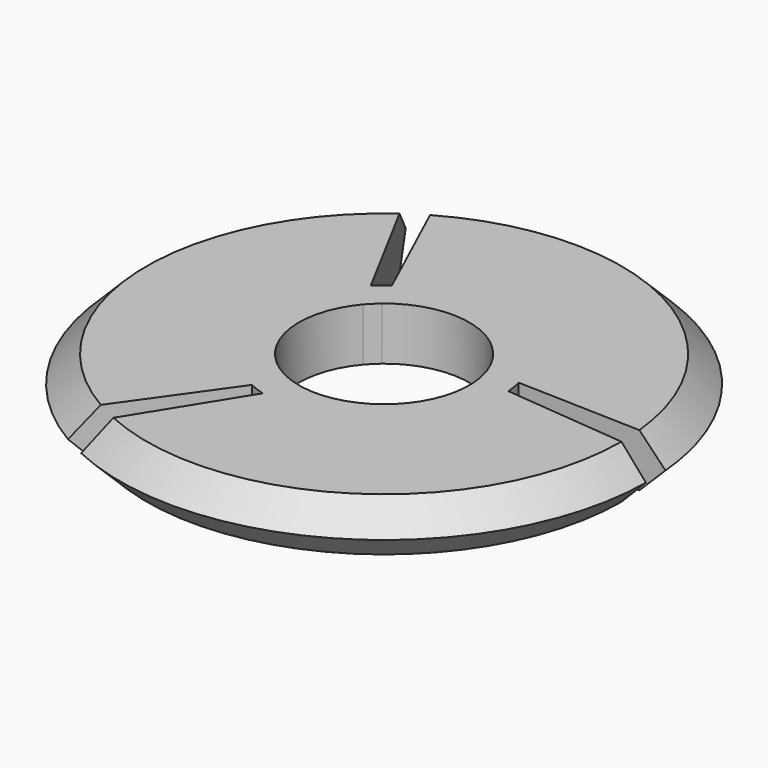
from build123d import *

# Parameters (mm, degrees)
F1_DEPTH     = 7
F2_T2_ANGLE  = 147.8228871573
F2_T4_ANGLE  = 147.8228871573
F2_T6_ANGLE  = 147.8228871573
F2_T8_ANGLE  = 147.8228871573
F2_T10_ANGLE = 147.8228871573
F2_T12_ANGLE = 147.8228871573


# Not quite as in the source:
# - a fillet or chamfer that OpenCascade refuses, or shapes differently, is made with other operations: its cross-section is extruded or revolved along the edge and cut away or added


with BuildPart() as f1:
    # F0 (on Top) → F1 (new body)
    with BuildSketch(Plane.XY):
        with BuildLine():
            Line((-28.4060324401, -36.6326823344), (-16.7057452382, -20.1458706432))
            ThreePointArc((-16.7057452382, -20.1458706432), (-25.4681782111, -8.7912963767), (-20.97968548, 4.8307453711))
            Line((-20.97968548, 4.8307453711), (-30.6144689612, 22.7902857677))
            ThreePointArc((-30.6144689612, 22.7902857677), (-45.7201890255, -7.5236357069), (-28.4060324401, -36.6326823344))
        make_face()
        with BuildLine():
            ThreePointArc((-19.29435824, 6.2304415143), (-5.0797919896, 8.1416439346), (4.4729958499, -2.5565256692))
            Line((4.4729958499, -2.5565256692), (24.8438058142, -3.1923286128))
            ThreePointArc((24.8438058142, -3.1923286128), (6.144039761, 25.0465694426), (-27.722212391, 24.6065933083))
            Line((-27.722212391, 24.6065933083), (-19.29435824, 6.2304415143))
        make_face()
        with BuildLine():
            ThreePointArc((4.9156669829, -6.2104463577), (-1.1968722093, -18.4456132191), (-14.6509092006, -20.9055587751))
            Line((-14.6509092006, -20.9055587751), (-25.3869356838, -38.229296228))
            ThreePointArc((-25.3869356838, -38.229296228), (8.4185504337, -36.154272809), (24.9706460004, -6.6052500471))
            Line((24.9706460004, -6.6052500471), (4.8425046474, -4.7159099443))
            ThreePointArc((4.8425046474, -4.7159099443), (4.8973654542, -5.4622833042), (4.9156669829, -6.2104463577))
        make_face()
        with BuildLine():
            Line((-16.7057452382, -20.1458706432), (-14.3009175091, -16.7572408399))
            ThreePointArc((-14.3009175091, -16.7572408399), (-21.2699622014, -9.0563128177), (-18.9622633915, 1.0702069463))
            Line((-18.9622633915, 1.0702069463), (-20.97968548, 4.8307453711))
            ThreePointArc((-20.97968548, 4.8307453711), (-25.4681782111, -8.7912963767), (-16.7057452382, -20.1458706432))
        make_face()
        with BuildLine():
            ThreePointArc((-17.5621326109, 2.4534847075), (-7.4084109648, 4.63839044), (0.2075629978, -2.4233952356))
            Line((0.2075629978, -2.4233952356), (4.4729958499, -2.5565256692))
            ThreePointArc((4.4729958499, -2.5565256692), (-5.0797919896, 8.1416439346), (-19.29435824, 6.2304415143))
            Line((-19.29435824, 6.2304415143), (-17.5621326109, 2.4534847075))
        make_face()
        with BuildLine():
            ThreePointArc((0.7054512892, -4.3275829408), (-2.4792256646, -14.2134166955), (-12.4028984371, -17.2781507839))
            Line((-12.4028984371, -17.2781507839), (-14.6509092006, -20.9055587751))
            ThreePointArc((-14.6509092006, -20.9055587751), (-1.1968722093, -18.4456132191), (4.9156669829, -6.2104463577))
            ThreePointArc((4.9156669829, -6.2104463577), (4.8973654542, -5.4622833042), (4.8425046474, -4.7159099443))
            Line((4.8425046474, -4.7159099443), (0.7054512892, -4.3275829408))
        make_face()
        with BuildLine():
            Line((-20.97968548, 4.8307453711), (-18.9622633915, 1.0702069463))
            ThreePointArc((-18.9622633915, 1.0702069463), (-18.2773306397, 1.7771628324), (-17.5621326109, 2.4534847075))
            Line((-17.5621326109, 2.4534847075), (-19.29435824, 6.2304415143))
            ThreePointArc((-19.29435824, 6.2304415143), (-20.1621039238, 5.5607939156), (-20.97968548, 4.8307453711))
        make_face()
        with BuildLine():
            ThreePointArc((0.2075629978, -2.4233952356), (0.4773383786, -3.3700423415), (0.7054512892, -4.3275829408))
            Line((0.7054512892, -4.3275829408), (4.8425046474, -4.7159099443))
            ThreePointArc((4.8425046474, -4.7159099443), (4.6964456573, -3.6295963387), (4.4729958499, -2.5565256692))
            Line((4.4729958499, -2.5565256692), (0.2075629978, -2.4233952356))
        make_face()
        with BuildLine():
            Line((-14.6509092006, -20.9055587751), (-12.4028984371, -17.2781507839))
            Line((-12.4028984371, -17.2781507839), (-14.3009175091, -16.7572408399))
            Line((-14.3009175091, -16.7572408399), (-16.7057452382, -20.1458706432))
            ThreePointArc((-16.7057452382, -20.1458706432), (-15.6919405642, -20.56253665), (-14.6509092006, -20.9055587751))
        make_face()
    extrude(amount=F1_DEPTH)

    # F2: chamfer of 4 on 6 edges, made by hand

    # F2_s1 → F2_t2 (revolve, cut)
    with BuildSketch(Plane(origin=(-11.2150452206, -3.6909975733, 0), x_dir=(0, 0, 1), z_dir=(0.9498795724, 0.3126160553, 0))):
        Polygon((3, -32.7063288851), (7, -28.7063288851), (7, -32.7063288851), align=None)
    revolve(axis=Axis((-10.3858662769, -6.2104463577, 7), (0, 0, 1)), revolution_arc=F2_T2_ANGLE, mode=Mode.SUBTRACT)

    # F2_s3 → F2_t4 (revolve, cut)
    with BuildSketch(Plane(origin=(-11.2150452206, -3.6909975733, 0), x_dir=(0, 0, 1), z_dir=(0.9498795724, 0.3126160553, 0))):
        Polygon((4, -32.7063288851), (0, -28.7063288851), (0, -32.7063288851), align=None)
    revolve(axis=Axis((-10.3858662769, -6.2104463577, 0), (0, 0, 1)), revolution_arc=F2_T4_ANGLE, mode=Mode.SUBTRACT)

    # F2_s5 → F2_t6 (revolve, cut)
    with BuildSketch(Plane(origin=(-2.6891726039, 2.4029660659, 0), x_dir=(0, 0, 1), z_dir=(-0.7456732317, 0.6663118126, 0))):
        Polygon((3, -46.9099054592), (7, -42.9099054592), (7, -46.9099054592), align=None)
    revolve(axis=Axis((-10.3858662769, -6.2104463577, 7), (0, 0, 1)), revolution_arc=F2_T6_ANGLE, mode=Mode.SUBTRACT)

    # F2_s7 → F2_t8 (revolve, cut)
    with BuildSketch(Plane(origin=(-2.6891726039, 2.4029660659, 0), x_dir=(0, 0, 1), z_dir=(-0.7456732317, 0.6663118126, 0))):
        Polygon((4, -46.9099054592), (0, -42.9099054592), (0, -46.9099054592), align=None)
    revolve(axis=Axis((-10.3858662769, -6.2104463577, 0), (0, 0, 1)), revolution_arc=F2_T8_ANGLE, mode=Mode.SUBTRACT)

    # F2_s9 → F2_t10 (revolve, cut)
    with BuildSketch(Plane(origin=(-1.6745815909, -8.0276380292, 0), x_dir=(0, 0, 1), z_dir=(-0.2042063407, -0.9789278678, 0))):
        Polygon((3, -26.4599150641), (7, -22.4599150641), (7, -26.4599150641), align=None)
    revolve(axis=Axis((-10.3858662769, -6.2104463577, 7), (0, 0, 1)), revolution_arc=F2_T10_ANGLE, mode=Mode.SUBTRACT)

    # F2_s11 → F2_t12 (revolve, cut)
    with BuildSketch(Plane(origin=(-1.6745815909, -8.0276380292, 0), x_dir=(0, 0, 1), z_dir=(-0.2042063407, -0.9789278678, 0))):
        Polygon((4, -26.4599150641), (0, -22.4599150641), (0, -26.4599150641), align=None)
    revolve(axis=Axis((-10.3858662769, -6.2104463577, 0), (0, 0, 1)), revolution_arc=F2_T12_ANGLE, mode=Mode.SUBTRACT)


solid = f1.part
